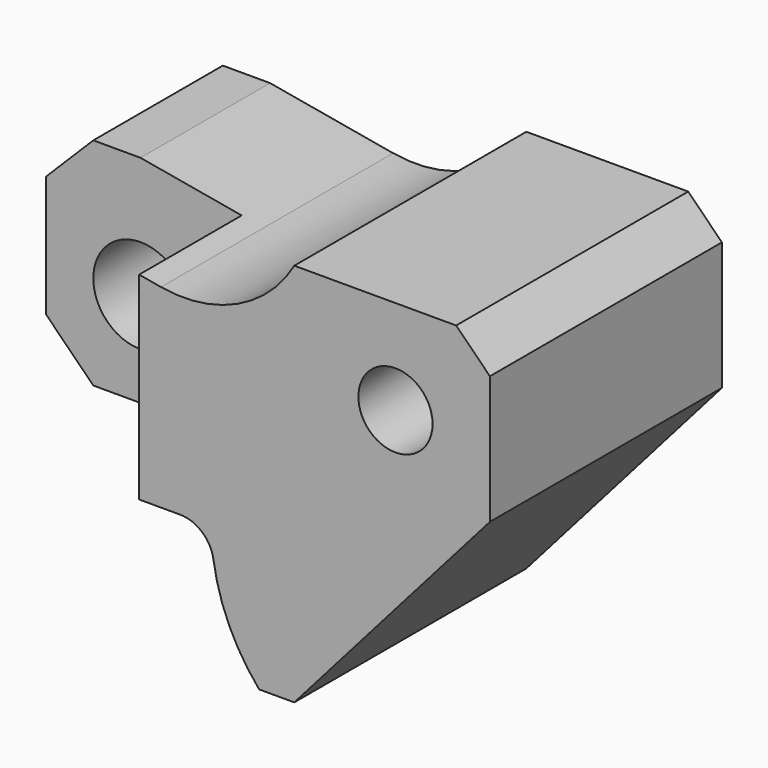
from build123d import *

# Parameters (mm, degrees)
F0_R     = 7
F1_DEPTH = 21.5
F2_R     = 5.5
F3_DEPTH = 43.001
F2_R_2   = 7
F4_DEPTH = 19


with BuildPart() as f1:
    # F0 (on Front) → F1 (new body, symmetric)
    with BuildSketch(Plane.XZ):
        with BuildLine():
            Line((-7, 18), (-14, 11))
            Line((-14, 11), (-14, -7))
            Line((-14, -7), (-7, -14))
            Line((-7, -14), (21.0666262554, -14))
            ThreePointArc((21.0666262554, -14), (24.3318620364, -15.2134137678), (26.0122649968, -18.2647058824))
            ThreePointArc((26.0122649968, -18.2647058824), (28.3490951999, -26.115672061), (32.7880673968, -33))
            Line((32.7880673968, -33), (38, -33))
            Line((38, -33), (67, 0))
            Line((67, 0), (67, 19))
            Line((67, 19), (62, 24))
            Line((62, 24), (38, 24))
            ThreePointArc((38, 24), (29.5749729609, 16.2760691513), (18.2430849879, 14.7832519053))
            Line((18.2430849879, 14.7832519053), (0, 18))
            Line((0, 18), (-7, 18))
        make_face()
        Circle(F0_R, mode=Mode.SUBTRACT)
    extrude(amount=F1_DEPTH, both=True)

    # F2 (on face) → F3 (cut, through all)
    with BuildSketch(Plane.XZ.offset(21.5)):
        with Locations((53, 10)):
            Circle(F2_R)
    extrude(amount=-F3_DEPTH, mode=Mode.SUBTRACT)

    # F2 (on face) → F4 (cut)
    with BuildSketch(Plane.XZ.offset(21.5)):
        Polygon((15, -14), (15, 15.3550952894), (0, 18), (-7, 18), (-14, 11), (-14, -7), (-7, -14), align=None)
        Circle(F2_R_2, mode=Mode.SUBTRACT)
    extrude(amount=-F4_DEPTH, mode=Mode.SUBTRACT)


solid = f1.part
